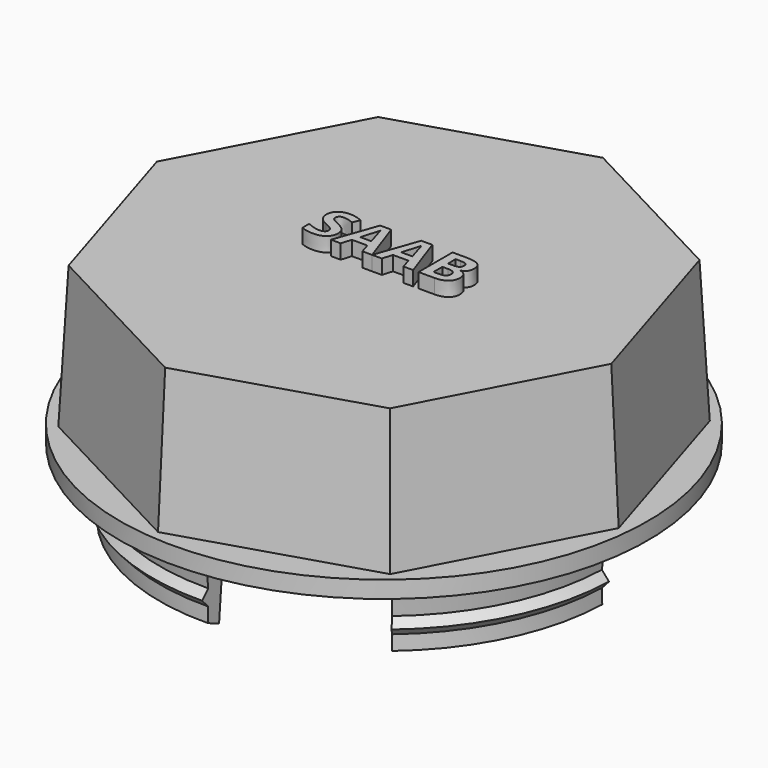
from build123d import *

# Parameters (mm, degrees)
F1_DEPTH     = 19.6
F1_TAPER     = 3
F6_R         = 29.5588051004
F7_DEPTH     = 17
F8_TEXT_SIZE = 8.2352567309
F9_DEPTH     = 2
F12_START    = -5
F12_DEPTH    = 20
F15_DEPTH    = 10


# Not quite as in the source:
# - the program builds the solid bodies; features that only make, move or delete a surface that nothing else refers to are left out
# - Text() gives the source's letters only with a copy of the font that has no kerning and outlines rounded to 1/6400 em; it was checked with that copy


with BuildPart() as f1:
    # F0 (on Top) → F1 (new body)
    with BuildSketch(Plane.XY):
        Polygon((6.846458452, 3.2292531715), (14.8228506263, -22.4859673376), (38.6464184239, -35.0292131433), (64.3616389329, -27.052820969), (76.9048847387, -3.2292531715), (68.9284925643, 22.4859673376), (45.1049247668, 35.0292131433), (19.3897042578, 27.052820969), align=None)
    extrude(amount=F1_DEPTH, taper=F1_TAPER)

    # F6 (on Top) → F7 (cut)
    with BuildSketch(Plane.XY):
        with Locations((41.8770387769, 0)):
            Circle(F6_R)
    extrude(amount=F7_DEPTH, mode=Mode.SUBTRACT)


with BuildPart() as f5:
    # F4 (on Front) → F5 (revolve)
    with BuildSketch(Plane.XZ):
        Polygon((12.6976181568, -12.3096757326), (13.6948058819, 0), (10.6566109201, 0), (5.3524481356, 0), (5.3524481356, -2.35), (10.3524481356, -2.35), (10.9037844754, -7.3195098592), (9.8944546766, -8.429128423), (10.9037844754, -9.5387469869), (10.8524481356, -11.5380880234), align=None)
    revolve(axis=Axis((41.8524481356, 0, -10.1716983277), (0, 0, -1)))


with BuildPart() as f9:
    # F8 (on Top) → F9 (new body)
    with BuildSketch(Plane.XY):
        with Locations((32.3866456747, -2.9817488976)):
            Text('SAAB', F8_TEXT_SIZE, font='Open Sans', font_style=FontStyle.BOLD, text_align=(TextAlign.LEFT, TextAlign.BOTTOM))
    extrude(amount=F9_DEPTH)


with BuildPart() as f9_1:
    # F10: moved
    add(f9.part.moved(Location((0, 0, 20))))


with BuildPart() as f12:
    # F11 (on Top) → F12 (new body)
    with BuildSketch(Plane.XY.offset(F12_START)):
        Polygon((42.6140986383, -43.1583486497), (69.8464736342, -34.131936729), (60.4310854986, -22.0097155725), (42.8283442474, -28.884228869), align=None)
        Polygon((42.8283442474, -28.884228869), (60.4310854986, -22.0097155725), (43.3466422396, -0.013660122), (43.260671187, -0.0804342567), align=None)
        Polygon((43.260671187, -0.0804342567), (43.3466422396, -0.013660122), (43.3372866763, -0.0016149246), (43.2618701985, -0.0005500774), align=None)
        Polygon((43.3372866763, -0.0016149246), (43.3466422396, -0.013660122), (43.3617063937, -0.0019597202), align=None)
        Polygon((43.2618701985, -0.0005500774), (43.3372866763, -0.0016149246), (43.2632842698, 0.093662458), align=None)
        Polygon((19.4793593917, -18.5514948023), (43.260671187, -0.0804342567), (43.2618701985, -0.0005500774), (43.2229116559, 0), (12.5911462439, 0.4803054209), align=None)
        Polygon((9.1356113553, -26.585534215), (19.4793593917, -18.5514948023), (12.5911462439, 0.4803054209), (0, 0.6777343224), align=None)
    extrude(amount=-F12_DEPTH)


with BuildPart() as f12b:
    # F11 (on Top) → F12, piece 2 (new body)
    with BuildSketch(Plane.XY.offset(F12_START)):
        Polygon((24.825832521, 23.8317032525), (43.2632842698, 0.093662458), (43.6881296354, 28.3989969936), align=None)
        Polygon((16.3248591125, 34.7766242921), (24.825832521, 23.8317032525), (43.6881296354, 28.3989969936), (43.9111739397, 43.2593300939), align=None)
    extrude(amount=-F12_DEPTH)


with BuildPart() as f12c:
    # F11 (on Top) → F12, piece 3 (new body)
    with BuildSketch(Plane.XY.offset(F12_START)):
        Polygon((65.2221173543, 16.9771278037), (43.3617063937, -0.0019597202), (71.1709585301, -0.3946140477), align=None)
        Polygon((79.0283353161, 27.7004844491), (65.2221173543, 16.9771278037), (71.1709585301, -0.3946140477), (86.5694135427, -0.6120334147), align=None)
    extrude(amount=-F12_DEPTH)


with BuildPart() as f5_1:
    add(f5.part)

    # F13: cut F12, F12c, F12b
    add(f12.part, mode=Mode.SUBTRACT)
    add(f12c.part, mode=Mode.SUBTRACT)
    add(f12b.part, mode=Mode.SUBTRACT)


with BuildPart() as f15:
    # F14 (on Top) → F15 (new body)
    with BuildSketch(Plane.XY):
        Polygon((81.2726734822, 21.7885523797), (76.6011070263, 26.0260878816), (43.354075402, 0), align=None)
    extrude(amount=-F15_DEPTH)


with BuildPart() as f15b:
    # F14 (on Top) → F15, piece 2 (new body)
    with BuildSketch(Plane.XY):
        Polygon((85.3246003462, 4.6040632222), (43.354075402, 0), (87.0625718818, -1.4589142), align=None)
    extrude(amount=-F15_DEPTH)


with BuildPart() as f15c:
    # F14 (on Top) → F15, piece 3 (new body)
    with BuildSketch(Plane.XY):
        Polygon((74.1051476533, -39.282963935), (43.354075402, 0), (69.7669919231, -45.9663748299), align=None)
    extrude(amount=-F15_DEPTH)


with BuildPart() as f15d:
    # F14 (on Top) → F15, piece 4 (new body)
    with BuildSketch(Plane.XY):
        Polygon((48.7939971237, -49.5901900761), (43.354075402, 0), (41.5855238111, -52.9851111108), align=None)
    extrude(amount=-F15_DEPTH)


with BuildPart() as f15e:
    # F14 (on Top) → F15, piece 5 (new body)
    with BuildSketch(Plane.XY):
        Polygon((5.9819950958, -29.2552146417), (43.354075402, 0), (1.6118744296, -23.9856476341), align=None)
    extrude(amount=-F15_DEPTH)


with BuildPart() as f15f:
    # F14 (on Top) → F15, piece 6 (new body)
    with BuildSketch(Plane.XY):
        Polygon((-3.8238455154, -5.1753017358), (43.354075402, 0), (-4.7618607516, 1.6060269319), align=None)
    extrude(amount=-F15_DEPTH)


with BuildPart() as f15g:
    # F14 (on Top) → F15, piece 7 (new body)
    with BuildSketch(Plane.XY):
        Polygon((14.7173287406, 36.5820182504), (43.354075402, 0), (20.0315345828, 40.5881967797), align=None)
    extrude(amount=-F15_DEPTH)


with BuildPart() as f15h:
    # F14 (on Top) → F15, piece 8 (new body)
    with BuildSketch(Plane.XY):
        Polygon((38.2881817991, 46.1805591199), (43.354075402, 0), (44.9157021402, 46.7857237843), align=None)
    extrude(amount=-F15_DEPTH)


with BuildPart() as f15g_1:
    # F16: moved
    add(f15g.part.moved(Location((0, 0, -2.35))))


with BuildPart() as f15f_1:
    # F16: moved
    add(f15f.part.moved(Location((0, 0, -2.35))))


with BuildPart() as f15e_1:
    # F16: moved
    add(f15e.part.moved(Location((0, 0, -2.35))))


with BuildPart() as f15d_1:
    # F16: moved
    add(f15d.part.moved(Location((0, 0, -2.35))))


with BuildPart() as f15c_1:
    # F16: moved
    add(f15c.part.moved(Location((0, 0, -2.35))))


with BuildPart() as f15b_1:
    # F16: moved
    add(f15b.part.moved(Location((0, 0, -2.35))))


with BuildPart() as f15_1:
    # F16: moved
    add(f15.part.moved(Location((0, 0, -2.35))))


with BuildPart() as f15h_1:
    # F16: moved
    add(f15h.part.moved(Location((0, 0, -2.35))))


with BuildPart() as f5_2:
    add(f5_1.part)

    # F17: cut F15g, F15f, F15e, F15d, F15c, F15b, F15, F15h
    add(f15g_1.part, mode=Mode.SUBTRACT)
    add(f15f_1.part, mode=Mode.SUBTRACT)
    add(f15e_1.part, mode=Mode.SUBTRACT)
    add(f15d_1.part, mode=Mode.SUBTRACT)
    add(f15c_1.part, mode=Mode.SUBTRACT)
    add(f15b_1.part, mode=Mode.SUBTRACT)
    add(f15_1.part, mode=Mode.SUBTRACT)
    add(f15h_1.part, mode=Mode.SUBTRACT)


solid = Compound([f1.part, f9_1.part, f5_2.part])
